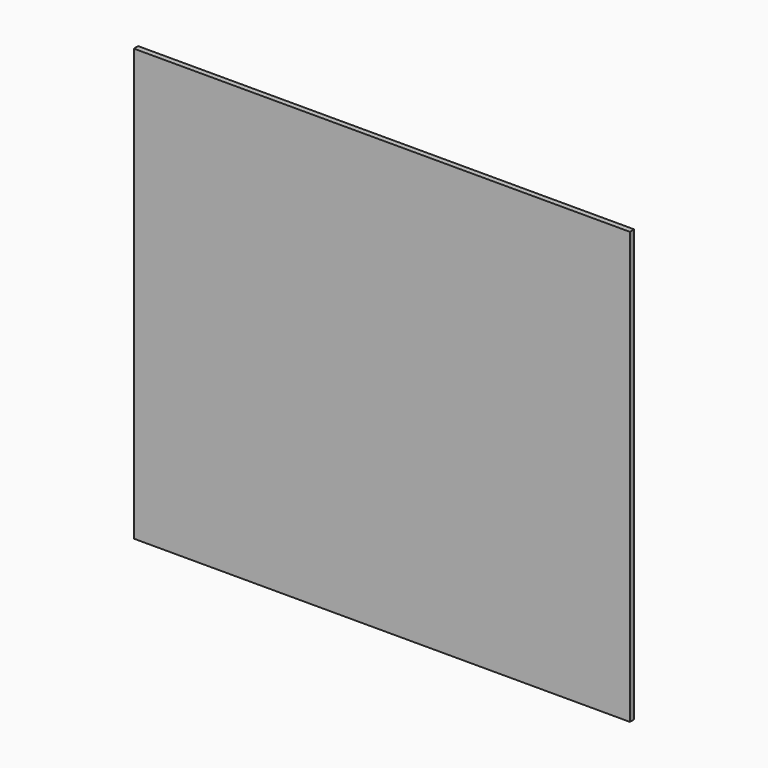
from build123d import *

# Parameters (mm, degrees)
F0_W     = 292.1
F0_H     = 254
F1_DEPTH = 3.175


# Not quite as in the source:
# - a length typed as a fraction of an inch, garbled in the dataset ("3 / 203.2 mm" for 3/8 in), is restored


with BuildPart() as f1:
    # F0 (on Front) → F1 (new body)
    with BuildSketch(Plane.XZ):
        Rectangle(F0_W, F0_H)
    extrude(amount=F1_DEPTH)


solid = f1.part
